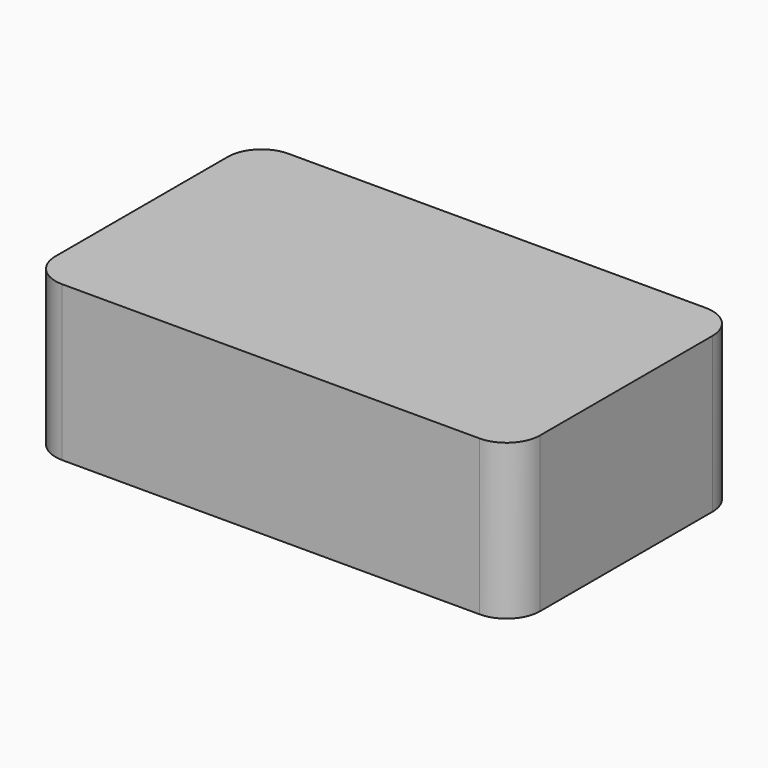
from build123d import *

# Parameters (mm, degrees)
F0_W     = 72
F0_H     = 42
F1_DEPTH = 23
F2_R     = 5
F3_T     = -1.9
F4_SIZE  = 0.8
F5_SIZE  = 1


with BuildPart() as f1:
    # F0 (on Top) → F1 (new body)
    with BuildSketch(Plane.XY):
        Rectangle(F0_W, F0_H)
    extrude(amount=F1_DEPTH)

    # F2
    f2_edges = [f1.edges().sort_by_distance(p)[0] for p in [
        (-36, -21, 11.5),
        (36, -21, 11.5),
        (36, 21, 11.5),
        (-36, 21, 11.5),
    ]]
    fillet(f2_edges, radius=F2_R)

    # F3
    f3_openings = [f1.faces().sort_by_distance(p)[0] for p in [
        (0, 0, 0),
    ]]
    offset(amount=F3_T, openings=f3_openings)

    # F4
    f4_edges = [f1.edges().sort_by_distance(p)[0] for p in [
        (34.1, 0, 0),
        (33.192031, -18.192031, 0),
        (0, -19.1, 0),
        (-33.192031, -18.192031, 0),
        (-34.1, 0, 0),
        (-33.192031, 18.192031, 0),
        (0, 19.1, 0),
        (33.192031, 18.192031, 0),
    ]]
    chamfer(f4_edges, length=F4_SIZE)

    # F5
    f5_edges = [f1.edges().sort_by_distance(p)[0] for p in [
        (34.1, 0, 21.1),
        (33.192031, 18.192031, 21.1),
        (0, 19.1, 21.1),
        (-33.192031, 18.192031, 21.1),
        (-34.1, 0, 21.1),
        (-33.192031, -18.192031, 21.1),
        (0, -19.1, 21.1),
        (33.192031, -18.192031, 21.1),
    ]]
    chamfer(f5_edges, length=F5_SIZE)

    # F7 (on offset) → F8 (revolve)
    with BuildSketch(Plane(origin=(0, 0, 4.5), x_dir=(1, 0, 0), z_dir=(0, 0, -1))):
        with BuildLine():
            Line((0, -19.1), (1.25, -19.1))
            ThreePointArc((1.25, -19.1), (0.8838834765, -18.2161165235), (0, -17.85))
            Line((0, -17.85), (0, -19.1))
        make_face()
        with BuildLine():
            Line((0, 19.1), (-1.25, 19.1))
            ThreePointArc((-1.25, 19.1), (-0.8838834765, 18.2161165235), (0, 17.85))
            Line((0, 17.85), (0, 19.1))
        make_face()
    revolve(axis=Axis((0, 18.475, 4.5), (0, 1, 0)))


solid = f1.part
